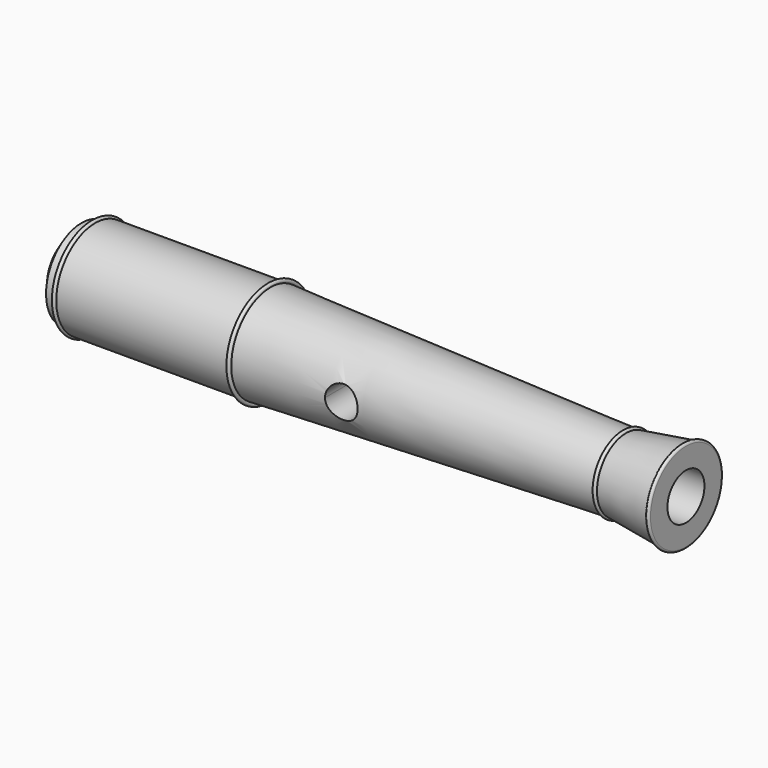
from build123d import *

# Parameters (mm, degrees)
F3_D     = 9.525
F3_DEPTH = 53.975
F3_TIP   = 2.861599
F5_D     = 6.5278
F5_DEPTH = 10.799373
F7_D     = 6.5278


with BuildPart() as f1:
    # F0 (on Front) → F1 (revolve)
    with BuildSketch(Plane.XZ):
        with BuildLine():
            Line((-34.136332, 0), (92.241368, 0))
            Line((92.241368, 0), (92.241368, 9.120069))
            ThreePointArc((92.241368, 9.120069), (91.847668, 9.513769), (91.453968, 9.120069))
            Line((91.453968, 9.120069), (79.935068, 7.501193))
            ThreePointArc((79.935068, 7.501193), (79.541368, 7.894893), (79.147668, 7.501193))
            Line((79.147668, 7.501193), (6.646209, 10.033))
            ThreePointArc((6.646209, 10.033), (6.516368, 10.798373), (6.386526, 10.033))
            Line((6.386526, 10.033), (-29.284932, 10.033))
            ThreePointArc((-29.284932, 10.033), (-29.678632, 10.4267), (-30.072332, 10.033))
            Line((-30.072332, 10.033), (-30.072332, 9.1313))
            Line((-30.072332, 9.1313), (-32.104332, 9.1313))
            Line((-32.104332, 9.1313), (-32.104332, 6.35))
            Line((-32.104332, 6.35), (-34.136332, 6.35))
            Line((-34.136332, 6.35), (-34.136332, 0))
        make_face()
    revolve(axis=Axis((29.052518, 0, 0), (-1, 0, 0)))

    # F3
    with Locations(Plane.YZ.offset(92.241368)):
        with Locations((0, 0)):
            Hole(F3_D / 2, depth=F3_DEPTH)
            with Locations((0, 0, -(F3_DEPTH + F3_TIP / 2))):  # 118° drill point
                Cone(0, F3_D / 2, F3_TIP, mode=Mode.SUBTRACT)

    # F5 (through all, one way)
    with BuildSketch(Plane(origin=(0, 0, 0), x_dir=(1, 0, 0), z_dir=(0, 1, 0))):
        with Locations((28.741368, 0)):
            Circle(F5_D / 2)
    extrude(amount=-F5_DEPTH, mode=Mode.SUBTRACT)

    # F7 (through all)
    with Locations(Plane.XZ):
        with Locations((28.741368, 0)):
            Hole(F7_D / 2)


solid = f1.part
